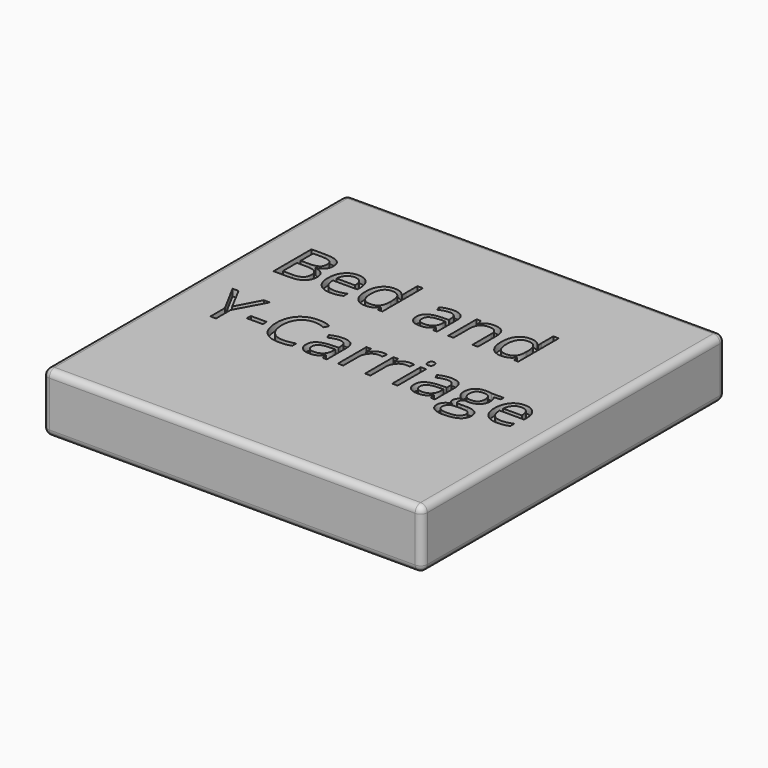
from build123d import *

# Parameters (mm, degrees)
F0_W         = 225
F0_H         = 225
F1_DEPTH     = 35
F2_R         = 4
F3_TEXT_SIZE = 39.4536192856
F4_DEPTH     = 4


# Not quite as in the source:
# - Text() gives the source's letters only with a copy of the font that has no kerning and outlines rounded to 1/6400 em; it was checked with that copy


with BuildPart() as f1:
    # F0 (on Top) → F1 (new body)
    with BuildSketch(Plane.XY):
        with Locations((-112.5, 112.5)):
            Rectangle(F0_W, F0_H)
    extrude(amount=F1_DEPTH)

    # F2
    f2_edges = [f1.edges().sort_by_distance(p)[0] for p in [
        (-225, 0, 17.5),
        (0, 0, 17.5),
        (-112.5, 0, 0),
        (-112.5, 0, 35),
        (0, 225, 17.5),
        (0, 112.5, 0),
        (0, 112.5, 35),
        (-112.5, 225, 35),
        (-225, 112.5, 35),
        (-225, 225, 17.5),
        (-225, 112.5, 0),
        (-112.5, 225, 0),
    ]]
    fillet(f2_edges, radius=F2_R)

    # F3 (on face) → F4 (cut)
    with BuildSketch(Plane.XY.offset(35)):
        with Locations((-206, 142.5933941144)):
            Text('Bed and', F3_TEXT_SIZE, font='Open Sans', text_align=(TextAlign.LEFT, TextAlign.BOTTOM))
        with Locations((-206, 88.9364718861)):
            Text('Y-Carriage', F3_TEXT_SIZE, font='Open Sans', text_align=(TextAlign.LEFT, TextAlign.BOTTOM))
    extrude(amount=-F4_DEPTH, mode=Mode.SUBTRACT)


solid = f1.part
